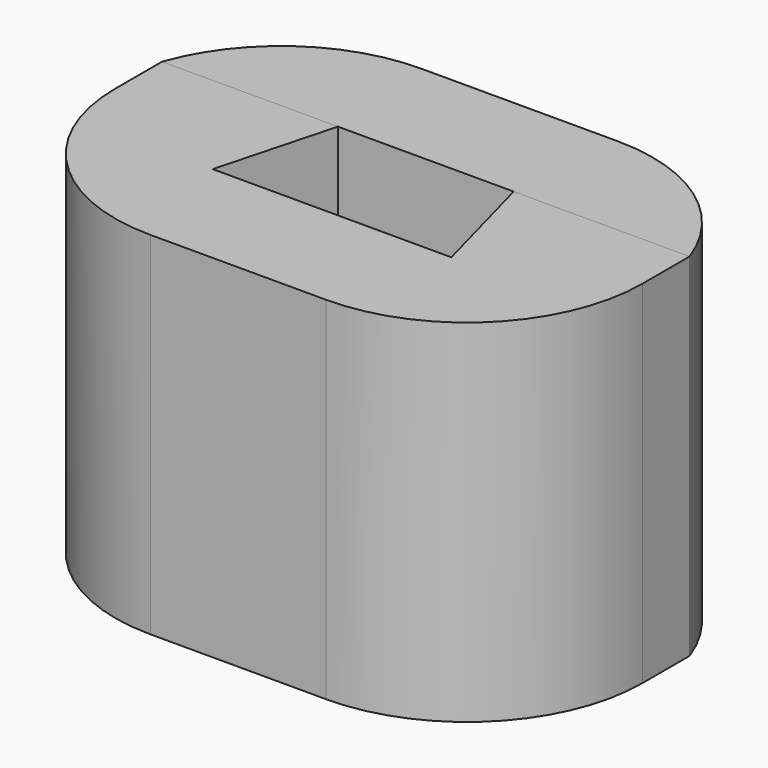
from build123d import *

# Parameters (mm, degrees)
F2_DEPTH      = 20
F3_DEPTH      = 20
F4_DEPTH      = 15
F5_DEPTH      = 5
F6_F1_R       = 10
F6_F2_R       = 10
F6_2_T1_DEPTH = 67.1404520791


# Not quite as in the source:
# - a fillet or chamfer that OpenCascade refuses, or shapes differently, is made with other operations: its cross-section is extruded or revolved along the edge and cut away or added


with BuildPart() as f2:
    # F1 (on Top) → F2 (new body)
    with BuildSketch(Plane.XY):
        Polygon((16.2058026315, -11.7642522434), (16.2058026315, 1.56908109), (6.2058026315, 1.56908109), (7.992130581, -5.0975855767), (1.2058026315, -5.0975855767), (-5.580525318, -5.0975855767), (-3.7941973685, 1.56908109), (-13.7941973685, 1.56908109), (-13.7941973685, -11.7642522434), align=None)
    extrude(amount=F2_DEPTH)

    # F1 (on Top) → F5 (join)
    with BuildSketch(Plane.XY):
        Polygon((5.980325855, 1.4446460496), (5.9469835864, 1.56908109), (1.2058026315, 1.56908109), (-3.5353783234, 1.56908109), (-3.568720592, 1.4446460496), (-5.2547189748, -4.8475855767), (-2.0442543917, -4.8475855767), (7.6663242378, -4.8475855767), align=None)
        Polygon((7.992130581, -5.0975855767), (6.2058026315, 1.56908109), (5.9469835864, 1.56908109), (5.980325855, 1.4446460496), (7.6663242378, -4.8475855767), (-2.0442543917, -4.8475855767), (-5.2547189748, -4.8475855767), (-3.568720592, 1.4446460496), (-3.5353783234, 1.56908109), (-3.7941973685, 1.56908109), (-5.580525318, -5.0975855767), (1.2058026315, -5.0975855767), align=None)
    extrude(amount=F5_DEPTH)

    # F6: fillet of radius 10 on 2 edges, made by hand

    # F6_f1
    f6_f1_edges = [f2.edges().sort_by_distance(p)[0] for p in [
        (16.2058026315, -11.7642522434, 10),
    ]]
    fillet(f6_f1_edges, radius=F6_F1_R)

    # F6_f2
    f6_f2_edges = [f2.edges().sort_by_distance(p)[0] for p in [
        (-13.7941973685, -11.7642522434, 10),
    ]]
    fillet(f6_f2_edges, radius=F6_F2_R)


with BuildPart() as f3:
    # F1 (on Top) → F3 (new body)
    with BuildSketch(Plane.XY):
        Polygon((6.2058026315, 1.56908109), (16.2058026315, 1.56908109), (16.2058026315, 8.2357477566), (-13.7941973685, 8.2357477566), (-13.7941973685, 1.56908109), (-3.7941973685, 1.56908109), (-3.5353783234, 1.56908109), (1.2058026315, 1.56908109), (5.9469835864, 1.56908109), align=None)
    extrude(amount=F3_DEPTH)

    # F1 (on Top) → F4 (join)
    with BuildSketch(Plane.XY):
        Polygon((5.980325855, 1.4446460496), (5.9469835864, 1.56908109), (1.2058026315, 1.56908109), (-3.5353783234, 1.56908109), (-3.568720592, 1.4446460496), (-5.2547189748, -4.8475855767), (-2.0442543917, -4.8475855767), (7.6663242378, -4.8475855767), align=None)
    extrude(amount=F4_DEPTH)

    # F6#2: fillet of radius 10 on 2 edges, made by hand

    # F6_2_s2 → F6_2_t1 (cut)
    with BuildSketch(Plane.XY.offset(-23.5702260396)):
        with BuildLine():
            ThreePointArc((-13.7941973685, 1.56908109), (-10.1396096446, 6.4007135659), (-4.3661069527, 8.2357477566))
            Line((-4.3661069527, 8.2357477566), (-13.7941973685, 8.2357477566))
            Line((-13.7941973685, 8.2357477566), (-13.7941973685, 1.56908109))
        make_face()
        with BuildLine():
            ThreePointArc((16.2058026315, 1.56908109), (12.5512149076, 6.4007135659), (6.7777122157, 8.2357477566))
            Line((6.7777122157, 8.2357477566), (16.2058026315, 8.2357477566))
            Line((16.2058026315, 8.2357477566), (16.2058026315, 1.56908109))
        make_face()
    extrude(amount=F6_2_T1_DEPTH, mode=Mode.SUBTRACT)


solid = Compound([f2.part, f3.part])
